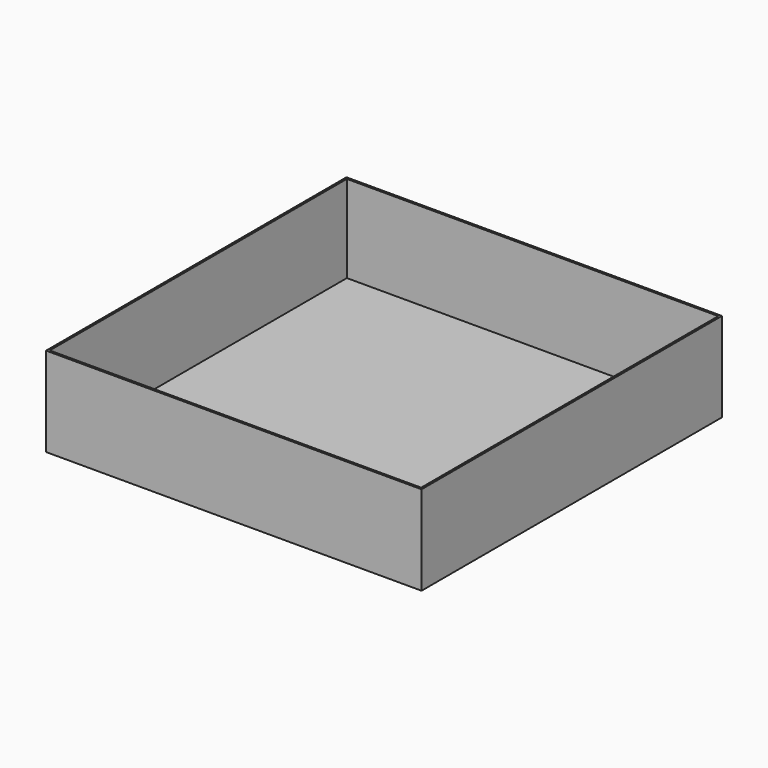
from build123d import *

# Parameters (mm, degrees)
F0_W     = 290.5125
F0_H     = 290.5125
F1_DEPTH = 1.5875
F2_W     = 293.6875
F2_H     = 293.6875
F2_W_2   = 290.5125
F2_H_2   = 290.5125
F3_DEPTH = 69.85


# Not quite as in the source:
# - a length typed as a fraction of an inch, garbled in the dataset ("3 / 203.2 mm" for 3/8 in), is restored


with BuildPart() as f1:
    # F0 (on Top) → F1 (new body)
    with BuildSketch(Plane.XY):
        with Locations((145.25625, 145.25625)):
            Rectangle(F0_W, F0_H)
    extrude(amount=F1_DEPTH)

    # F2 (on face) → F3 (join)
    with BuildSketch(Plane(origin=(0, 0, 0), x_dir=(1, 0, 0), z_dir=(0, 0, -1))):
        with Locations((145.25625, -145.25625)):
            Rectangle(F2_W, F2_H)
        with Locations((145.25625, -145.25625)):
            Rectangle(F2_W_2, F2_H_2, mode=Mode.SUBTRACT)
    extrude(amount=-F3_DEPTH)


solid = f1.part
